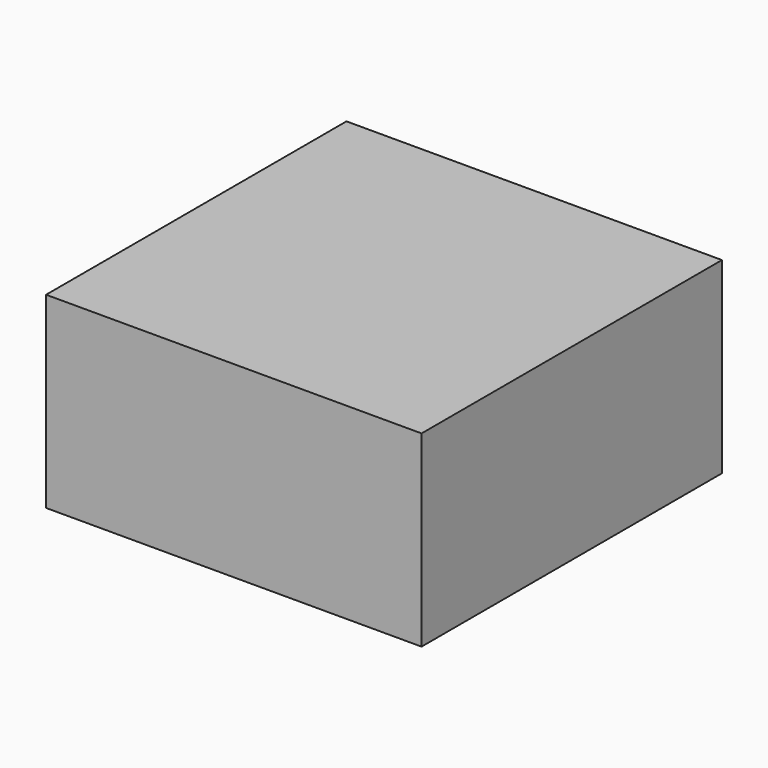
from build123d import *

# Parameters (mm, degrees)
F0_W     = 1000
F0_H     = 1000
F1_DEPTH = 500
F2_W     = 940
F2_H     = 940
F3_DEPTH = 10
F4_T     = -1.5


# Not quite as in the source:
# - a shell that OpenCascade refuses in one call is made with other operations: the cavity is built on its own and cut out


with BuildPart() as f1:
    # F0 (on Top) → F1 (new body)
    with BuildSketch(Plane.XY):
        Rectangle(F0_W, F0_H)
    extrude(amount=F1_DEPTH)

    # F2 (on face) → F3 (cut)
    with BuildSketch(Plane(origin=(0, 0, 0), x_dir=(1, 0, 0), z_dir=(0, 0, -1))):
        Rectangle(F2_W, F2_H)
    extrude(amount=-F3_DEPTH, mode=Mode.SUBTRACT)

    # F4: a shell. OpenCascade refuses it in one call, so the cavity is built on its own and cut out:
    # the body offset inwards by the wall thickness, plus a prism from it out through each open face.
    f4_core = offset(f1.part, amount=F4_T, kind=Kind.INTERSECTION, mode=Mode.PRIVATE)
    f4_exits = [f4_core.faces().sort_by_distance(p)[0] for p in [
        (0, 0, 11.5),
    ]]
    add(f4_core, mode=Mode.SUBTRACT)
    extrude(f4_exits, amount=-F4_T, mode=Mode.SUBTRACT)


solid = f1.part
